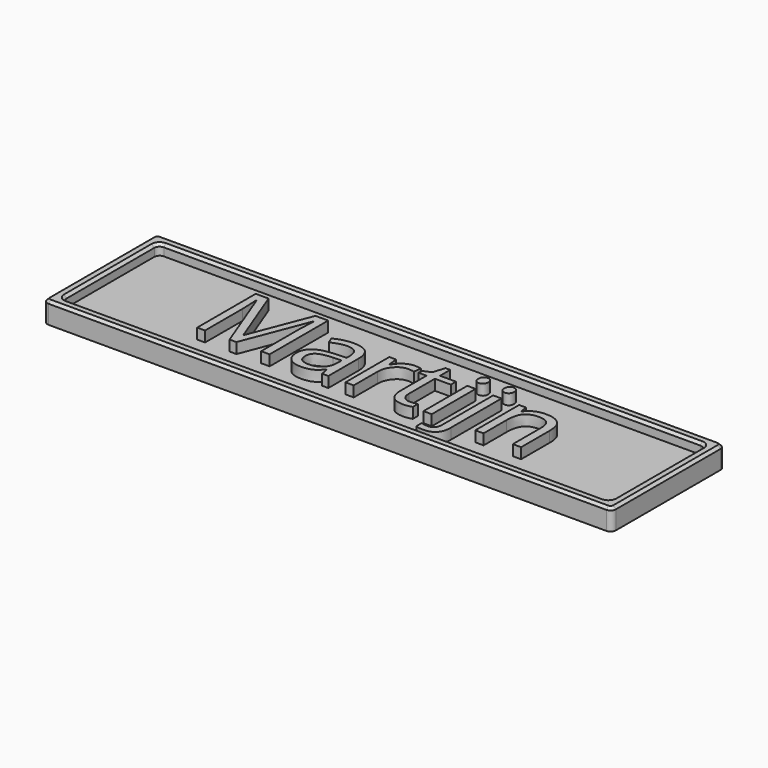
from build123d import *

# Parameters (mm, degrees)
F1_DEPTH     = 4
F0_TEXT_SIZE = 19.3397863768
F2_DEPTH     = 4
F0_W         = 1.5683358015
F0_H         = 10.3498075532
F3_DEPTH     = 2
F4_SIZE      = 0.5


# Not quite as in the source:
# - Text() gives the source's letters only with a copy of the font that has no kerning and outlines rounded to 1/6400 em; it was checked with that copy


with BuildPart() as f1:
    # F0 (on Top) → F1 (new body)
    with BuildSketch(Plane.XY):
        with BuildLine():
            Line((-52.6345206201, -13.340712525), (52.6345206201, -13.340712525))
            ThreePointArc((52.6345206201, -13.340712525), (53.3416274013, -13.0478193061), (53.6345206201, -12.340712525))
            Line((53.6345206201, -12.340712525), (53.6345206201, 12.340712525))
            ThreePointArc((53.6345206201, 12.340712525), (53.3416274013, 13.0478193061), (52.6345206201, 13.340712525))
            Line((52.6345206201, 13.340712525), (32.1950025846, 13.340712525))
            Line((32.1950025846, 13.340712525), (-52.6345206201, 13.340712525))
            ThreePointArc((-52.6345206201, 13.340712525), (-53.3416274013, 13.0478193061), (-53.6345206201, 12.340712525))
            Line((-53.6345206201, 12.340712525), (-53.6345206201, -12.340712525))
            ThreePointArc((-53.6345206201, -12.340712525), (-53.3416274013, -13.0478193061), (-52.6345206201, -13.340712525))
        make_face()
        with BuildLine():
            Line((-50.6345206201, 11.340712525), (50.6345206201, 11.340712525))
            ThreePointArc((50.6345206201, 11.340712525), (51.3416274013, 11.0478193061), (51.6345206201, 10.340712525))
            Line((51.6345206201, 10.340712525), (51.6345206201, -10.340712525))
            ThreePointArc((51.6345206201, -10.340712525), (51.3416274013, -11.0478193061), (50.6345206201, -11.340712525))
            Line((50.6345206201, -11.340712525), (-50.6345206201, -11.340712525))
            ThreePointArc((-50.6345206201, -11.340712525), (-51.3416274013, -11.0478193061), (-51.6345206201, -10.340712525))
            Line((-51.6345206201, -10.340712525), (-51.6345206201, 10.340712525))
            ThreePointArc((-51.6345206201, 10.340712525), (-51.3416274013, 11.0478193061), (-50.6345206201, 11.340712525))
        make_face(mode=Mode.SUBTRACT)
    extrude(amount=F1_DEPTH)



with BuildPart() as f2:
    # F0 (on Top) → F2 (new body)
    with BuildSketch(Plane.XY):
        with Locations((-32.0946779102, -6.3302232884)):
            Text('Martijn', F0_TEXT_SIZE, font='Open Sans', text_align=(TextAlign.LEFT, TextAlign.BOTTOM))
    extrude(amount=F2_DEPTH)


with BuildPart() as f1_1:
    add(f1.part)

    add(f2.part)  # F3 merges F2
    # F0 (on Top) → F3 (join)
    with BuildSketch(Plane.XY):
        with BuildLine():
            ThreePointArc((51.6345206201, 10.340712525), (51.3416274013, 11.0478193061), (50.6345206201, 11.340712525))
            Line((50.6345206201, 11.340712525), (-50.6345206201, 11.340712525))
            ThreePointArc((-50.6345206201, 11.340712525), (-51.3416274013, 11.0478193061), (-51.6345206201, 10.340712525))
            Line((-51.6345206201, 10.340712525), (-51.6345206201, -10.340712525))
            ThreePointArc((-51.6345206201, -10.340712525), (-51.3416274013, -11.0478193061), (-50.6345206201, -11.340712525))
            Line((-50.6345206201, -11.340712525), (50.6345206201, -11.340712525))
            ThreePointArc((50.6345206201, -11.340712525), (51.3416274013, -11.0478193061), (51.6345206201, -10.340712525))
            Line((51.6345206201, -10.340712525), (51.6345206201, 10.340712525))
        make_face()
        with BuildLine():
            Line((-5.4450566513, -6.3302232884), (-6.6084656755, -6.3302232884))
            Line((-6.6084656755, -6.3302232884), (-6.9197153625, -4.8555645772))
            Line((-6.9197153625, -4.8555645772), (-6.9952614031, -4.8555645772))
            add(Edge.make_bspline(
                [(-6.9952614031, -4.8555645772), (-7.7688528581, -5.8285975792), (-8.5379115508, -6.1745984449)],
                knots=[0, 0, 0, 1, 1, 1], degree=2))
            add(Edge.make_bspline(
                [(-8.5379115508, -6.1745984449), (-9.3069702434, -6.5205993105), (-10.4613137428, -6.5205993105)],
                knots=[0, 0, 0, 1, 1, 1], degree=2))
            add(Edge.make_bspline(
                [(-10.4613137428, -6.5205993105), (-11.9994311281, -6.5205993105), (-12.8727433566, -5.7258549641)],
                knots=[0, 0, 0, 1, 1, 1], degree=2))
            add(Edge.make_bspline(
                [(-12.8727433566, -5.7258549641), (-13.7460555852, -4.9311106177), (-13.7460555852, -3.4685392729)],
                knots=[0, 0, 0, 1, 1, 1], degree=2))
            add(Edge.make_bspline(
                [(-13.7460555852, -3.4685392729), (-13.7460555852, -0.3348895116), (-8.7328203354, -0.1837974305)],
                knots=[0, 0, 0, 1, 1, 1], degree=2))
            Line((-8.7328203354, -0.1837974305), (-6.9771303533, -0.1263824397))
            Line((-6.9771303533, -0.1263824397), (-6.9771303533, 0.5172698257))
            add(Edge.make_bspline(
                [(-6.9771303533, 0.5172698257), (-6.9771303533, 1.7350719991), (-7.4999089538, 2.3152655904)],
                knots=[0, 0, 0, 1, 1, 1], degree=2))
            add(Edge.make_bspline(
                [(-7.4999089538, 2.3152655904), (-8.0226875543, 2.8954591817), (-9.1770310537, 2.8954591817)],
                knots=[0, 0, 0, 1, 1, 1], degree=2))
            add(Edge.make_bspline(
                [(-9.1770310537, 2.8954591817), (-10.4703792676, 2.8954591817), (-12.1021737432, 2.1037366769)],
                knots=[0, 0, 0, 1, 1, 1], degree=2))
            Line((-12.1021737432, 2.1037366769), (-12.5856684026, 3.3034078006))
            add(Edge.make_bspline(
                [(-12.5856684026, 3.3034078006), (-11.8211424724, 3.7174001027), (-10.9100572236, 3.9531037492)],
                knots=[0, 0, 0, 1, 1, 1], degree=2))
            add(Edge.make_bspline(
                [(-10.9100572236, 3.9531037492), (-9.9989719747, 4.1888073956), (-9.0803321218, 4.1888073956)],
                knots=[0, 0, 0, 1, 1, 1], degree=2))
            add(Edge.make_bspline(
                [(-9.0803321218, 4.1888073956), (-7.2309650495, 4.1888073956), (-6.3380108504, 3.3683773954)],
                knots=[0, 0, 0, 1, 1, 1], degree=2))
            add(Edge.make_bspline(
                [(-6.3380108504, 3.3683773954), (-5.4450566513, 2.5479473952), (-5.4450566513, 0.7348424224)],
                knots=[0, 0, 0, 1, 1, 1], degree=2))
            Line((-5.4450566513, 0.7348424224), (-5.4450566513, -6.3302232884))
        make_face(mode=Mode.SUBTRACT)
        with BuildLine():
            add(Edge.make_bspline(
                [(18.9653799662, -7.9166901396), (18.9653799662, -10.9778157021), (16.1399580502, -10.9778157021)],
                knots=[0, 0, 0, 1, 1, 1], degree=2))
            add(Edge.make_bspline(
                [(16.1399580502, -10.9778157021), (15.2424710886, -10.9778157021), (14.6864522303, -10.739090214)],
                knots=[0, 0, 0, 1, 1, 1], degree=2))
            Line((14.6864522303, -10.739090214), (14.6864522303, -9.4668948914))
            add(Edge.make_bspline(
                [(14.6864522303, -9.4668948914), (15.3391700205, -9.6542490719), (15.9707349194, -9.6542490719)],
                knots=[0, 0, 0, 1, 1, 1], degree=2))
            add(Edge.make_bspline(
                [(15.9707349194, -9.6542490719), (16.708064275, -9.6542490719), (17.0525542198, -9.2523441363)],
                knots=[0, 0, 0, 1, 1, 1], degree=2))
            add(Edge.make_bspline(
                [(17.0525542198, -9.2523441363), (17.3970441647, -8.8504392006), (17.3970441647, -8.0315201212)],
                knots=[0, 0, 0, 1, 1, 1], degree=2))
            Line((17.3970441647, -8.0315201212), (17.3970441647, 4.0195842648))
            Line((17.3970441647, 4.0195842648), (18.9653799662, 4.0195842648))
            Line((18.9653799662, 4.0195842648), (18.9653799662, -7.9166901396))
        make_face(mode=Mode.SUBTRACT)
        with BuildLine():
            add(Edge.make_bspline(
                [(0.7195002563, 3.6614960327), (1.5323756525, 4.209960287), (2.5054086545, 4.209960287)],
                knots=[0, 0, 0, 1, 1, 1], degree=2))
            add(Edge.make_bspline(
                [(2.5054086545, 4.209960287), (3.1943885442, 4.209960287), (3.7413418777, 4.0951303054)],
                knots=[0, 0, 0, 1, 1, 1], degree=2))
            Line((3.7413418777, 4.0951303054), (3.5237692809, 2.6416244855))
            add(Edge.make_bspline(
                [(3.5237692809, 2.6416244855), (2.8831388572, 2.7836510417), (2.3905786729, 2.7836510417)],
                knots=[0, 0, 0, 1, 1, 1], degree=2))
            add(Edge.make_bspline(
                [(2.3905786729, 2.7836510417), (1.1334925584, 2.7836510417), (0.2420492801, 1.7637794945)],
                knots=[0, 0, 0, 1, 1, 1], degree=2))
            add(Edge.make_bspline(
                [(0.2420492801, 1.7637794945), (-0.6493939982, 0.7439079473), (-0.6493939982, -0.7760783883)],
                knots=[0, 0, 0, 1, 1, 1], degree=2))
            Line((-0.6493939982, -0.7760783883), (-0.6493939982, -6.3302232884))
            Line((-0.6493939982, -6.3302232884), (-2.2177297997, -6.3302232884))
            Line((-2.2177297997, -6.3302232884), (-2.2177297997, 4.0195842648))
            Line((-2.2177297997, 4.0195842648), (-0.9243815857, 4.0195842648))
            Line((-0.9243815857, 4.0195842648), (-0.7430710884, 2.1037366769))
            Line((-0.7430710884, 2.1037366769), (-0.6675250479, 2.1037366769))
            add(Edge.make_bspline(
                [(-0.6675250479, 2.1037366769), (-0.0933751398, 3.1130317784), (0.7195002563, 3.6614960327)],
                knots=[0, 0, 0, 1, 1, 1], degree=2))
        make_face(mode=Mode.SUBTRACT)
        with Locations((13.2888504804, -1.1553195118)):
            Rectangle(F0_W, F0_H, mode=Mode.SUBTRACT)
        with BuildLine():
            add(Edge.make_bspline(
                [(7.8026970168, -4.7241144666), (8.2469077352, -5.224229255), (9.0204991902, -5.224229255)],
                knots=[0, 0, 0, 1, 1, 1], degree=2))
            add(Edge.make_bspline(
                [(9.0204991902, -5.224229255), (9.437513334, -5.224229255), (9.8243090615, -5.1637924225)],
                knots=[0, 0, 0, 1, 1, 1], degree=2))
            add(Edge.make_bspline(
                [(9.8243090615, -5.1637924225), (10.2111047891, -5.1033555901), (10.4377429107, -5.0368750744)],
                knots=[0, 0, 0, 1, 1, 1], degree=2))
            Line((10.4377429107, -5.0368750744), (10.4377429107, -6.2365461981))
            add(Edge.make_bspline(
                [(10.4377429107, -6.2365461981), (10.1839082145, -6.357419863), (9.6883261886, -6.4390095868)],
                knots=[0, 0, 0, 1, 1, 1], degree=2))
            add(Edge.make_bspline(
                [(9.6883261886, -6.4390095868), (9.1927441626, -6.5205993105), (8.7938610686, -6.5205993105)],
                knots=[0, 0, 0, 1, 1, 1], degree=2))
            add(Edge.make_bspline(
                [(8.7938610686, -6.5205993105), (5.7931723386, -6.5205993105), (5.7931723386, -3.356731133)],
                knots=[0, 0, 0, 1, 1, 1], degree=2))
            Line((5.7931723386, -3.356731133), (5.7931723386, 2.8017820914))
            Line((5.7931723386, 2.8017820914), (4.3094481025, 2.8017820914))
            Line((4.3094481025, 2.8017820914), (4.3094481025, 3.5572424968))
            Line((4.3094481025, 3.5572424968), (5.7931723386, 4.209960287))
            Line((5.7931723386, 4.209960287), (6.4519338121, 6.4189265122))
            Line((6.4519338121, 6.4189265122), (7.3584862985, 6.4189265122))
            Line((7.3584862985, 6.4189265122), (7.3584862985, 4.0195842648))
            Line((7.3584862985, 4.0195842648), (10.3621968701, 4.0195842648))
            Line((10.3621968701, 4.0195842648), (10.3621968701, 2.8017820914))
            Line((10.3621968701, 2.8017820914), (7.3584862985, 2.8017820914))
            Line((7.3584862985, 2.8017820914), (7.3584862985, -3.2902506173))
            add(Edge.make_bspline(
                [(7.3584862985, -3.2902506173), (7.3584862985, -4.2239996783), (7.8026970168, -4.7241144666)],
                knots=[0, 0, 0, 1, 1, 1], degree=2))
        make_face(mode=Mode.SUBTRACT)
        with BuildLine():
            Line((30.9409383117, -6.3302232884), (29.3726025102, -6.3302232884))
            Line((29.3726025102, -6.3302232884), (29.3726025102, 0.3661777446))
            add(Edge.make_bspline(
                [(29.3726025102, 0.3661777446), (29.3726025102, 1.6293075423), (28.7969416813, 2.2533178371)],
                knots=[0, 0, 0, 1, 1, 1], degree=2))
            add(Edge.make_bspline(
                [(28.7969416813, 2.2533178371), (28.2212808524, 2.8773281319), (26.9913913125, 2.8773281319)],
                knots=[0, 0, 0, 1, 1, 1], degree=2))
            add(Edge.make_bspline(
                [(26.9913913125, 2.8773281319), (25.3686623619, 2.8773281319), (24.6132019565, 1.9994831409)],
                knots=[0, 0, 0, 1, 1, 1], degree=2))
            add(Edge.make_bspline(
                [(24.6132019565, 1.9994831409), (23.8577415512, 1.1216381499), (23.8577415512, -0.8999738948)],
                knots=[0, 0, 0, 1, 1, 1], degree=2))
            Line((23.8577415512, -0.8999738948), (23.8577415512, -6.3302232884))
            Line((23.8577415512, -6.3302232884), (22.2894057497, -6.3302232884))
            Line((22.2894057497, -6.3302232884), (22.2894057497, 4.0195842648))
            Line((22.2894057497, 4.0195842648), (23.5646229139, 4.0195842648))
            Line((23.5646229139, 4.0195842648), (23.8184576101, 2.6023405444))
            Line((23.8184576101, 2.6023405444), (23.8940036506, 2.6023405444))
            add(Edge.make_bspline(
                [(23.8940036506, 2.6023405444), (24.3774983101, 3.3668664746), (25.2462777762, 3.7884133808)],
                knots=[0, 0, 0, 1, 1, 1], degree=2))
            add(Edge.make_bspline(
                [(25.2462777762, 3.7884133808), (26.1150572424, 4.209960287), (27.1817673347, 4.209960287)],
                knots=[0, 0, 0, 1, 1, 1], degree=2))
            add(Edge.make_bspline(
                [(27.1817673347, 4.209960287), (29.0522872983, 4.209960287), (29.996612805, 3.307940563)],
                knots=[0, 0, 0, 1, 1, 1], degree=2))
            add(Edge.make_bspline(
                [(29.996612805, 3.307940563), (30.9409383117, 2.405920839), (30.9409383117, 0.4205708938)],
                knots=[0, 0, 0, 1, 1, 1], degree=2))
            Line((30.9409383117, 0.4205708938), (30.9409383117, -6.3302232884))
        make_face(mode=Mode.SUBTRACT)
        with BuildLine():
            Line((-22.7934493996, -6.3302232884), (-24.0867976136, -6.3302232884))
            Line((-24.0867976136, -6.3302232884), (-28.7706521267, 5.9082352782))
            Line((-28.7706521267, 5.9082352782), (-28.8461981672, 5.9082352782))
            add(Edge.make_bspline(
                [(-28.8461981672, 5.9082352782), (-28.7132371359, 4.4547294583), (-28.7132371359, 2.4512484633)],
                knots=[0, 0, 0, 1, 1, 1], degree=2))
            Line((-28.7132371359, 2.4512484633), (-28.7132371359, -6.3302232884))
            Line((-28.7132371359, -6.3302232884), (-30.196961372, -6.3302232884))
            Line((-30.196961372, -6.3302232884), (-30.196961372, 7.4765710797))
            Line((-30.196961372, 7.4765710797), (-27.7794880749, 7.4765710797))
            Line((-27.7794880749, 7.4765710797), (-23.4068832488, -3.9127499913))
            Line((-23.4068832488, -3.9127499913), (-23.3313372082, -3.9127499913))
            Line((-23.3313372082, -3.9127499913), (-18.9224702826, 7.4765710797))
            Line((-18.9224702826, 7.4765710797), (-16.5231280353, 7.4765710797))
            Line((-16.5231280353, 7.4765710797), (-16.5231280353, -6.3302232884))
            Line((-16.5231280353, -6.3302232884), (-18.1277259362, -6.3302232884))
            Line((-18.1277259362, -6.3302232884), (-18.1277259362, 2.5660784449))
            add(Edge.make_bspline(
                [(-18.1277259362, 2.5660784449), (-18.1277259362, 4.0951303054), (-17.9947649049, 5.8901042285)],
                knots=[0, 0, 0, 1, 1, 1], degree=2))
            Line((-17.9947649049, 5.8901042285), (-18.0703109454, 5.8901042285))
            Line((-18.0703109454, 5.8901042285), (-22.7934493996, -6.3302232884))
        make_face(mode=Mode.SUBTRACT)
        with BuildLine():
            add(Edge.make_bspline(
                [(12.6361326902, 6.0351526263), (12.3717215483, 6.2950310057), (12.3717215483, 6.8238532895)],
                knots=[0, 0, 0, 1, 1, 1], degree=2))
            add(Edge.make_bspline(
                [(12.3717215483, 6.8238532895), (12.3717215483, 7.3617410981), (12.6361326902, 7.6125539526)],
                knots=[0, 0, 0, 1, 1, 1], degree=2))
            add(Edge.make_bspline(
                [(12.6361326902, 7.6125539526), (12.9005438321, 7.8633668072), (13.2994269261, 7.8633668072)],
                knots=[0, 0, 0, 1, 1, 1], degree=2))
            add(Edge.make_bspline(
                [(13.2994269261, 7.8633668072), (13.6771571288, 7.8633668072), (13.9506337955, 7.6080211902)],
                knots=[0, 0, 0, 1, 1, 1], degree=2))
            add(Edge.make_bspline(
                [(13.9506337955, 7.6080211902), (14.2241104622, 7.3526755732), (14.2241104622, 6.8238532895)],
                knots=[0, 0, 0, 1, 1, 1], degree=2))
            add(Edge.make_bspline(
                [(14.2241104622, 6.8238532895), (14.2241104622, 6.2950310057), (13.9506337955, 6.0351526263)],
                knots=[0, 0, 0, 1, 1, 1], degree=2))
            add(Edge.make_bspline(
                [(13.9506337955, 6.0351526263), (13.6771571288, 5.7752742468), (13.2994269261, 5.7752742468)],
                knots=[0, 0, 0, 1, 1, 1], degree=2))
            add(Edge.make_bspline(
                [(13.2994269261, 5.7752742468), (12.9005438321, 5.7752742468), (12.6361326902, 6.0351526263)],
                knots=[0, 0, 0, 1, 1, 1], degree=2))
        make_face(mode=Mode.SUBTRACT)
        with BuildLine():
            add(Edge.make_bspline(
                [(17.5284942752, 6.0351526263), (17.2640831333, 6.2950310057), (17.2640831333, 6.8238532895)],
                knots=[0, 0, 0, 1, 1, 1], degree=2))
            add(Edge.make_bspline(
                [(17.2640831333, 6.8238532895), (17.2640831333, 7.3617410981), (17.5284942752, 7.6125539526)],
                knots=[0, 0, 0, 1, 1, 1], degree=2))
            add(Edge.make_bspline(
                [(17.5284942752, 7.6125539526), (17.7929054171, 7.8633668072), (18.1917885111, 7.8633668072)],
                knots=[0, 0, 0, 1, 1, 1], degree=2))
            add(Edge.make_bspline(
                [(18.1917885111, 7.8633668072), (18.5695187138, 7.8633668072), (18.8429953805, 7.6080211902)],
                knots=[0, 0, 0, 1, 1, 1], degree=2))
            add(Edge.make_bspline(
                [(18.8429953805, 7.6080211902), (19.1164720472, 7.3526755732), (19.1164720472, 6.8238532895)],
                knots=[0, 0, 0, 1, 1, 1], degree=2))
            add(Edge.make_bspline(
                [(19.1164720472, 6.8238532895), (19.1164720472, 6.2950310057), (18.8429953805, 6.0351526263)],
                knots=[0, 0, 0, 1, 1, 1], degree=2))
            add(Edge.make_bspline(
                [(18.8429953805, 6.0351526263), (18.5695187138, 5.7752742468), (18.1917885111, 5.7752742468)],
                knots=[0, 0, 0, 1, 1, 1], degree=2))
            add(Edge.make_bspline(
                [(18.1917885111, 5.7752742468), (17.7929054171, 5.7752742468), (17.5284942752, 6.0351526263)],
                knots=[0, 0, 0, 1, 1, 1], degree=2))
        make_face(mode=Mode.SUBTRACT)
        with BuildLine():
            add(Edge.make_bspline(
                [(-11.5884606676, -4.7815294574), (-11.0747475919, -5.224229255), (-10.1500640558, -5.224229255)],
                knots=[0, 0, 0, 1, 1, 1], degree=2))
            add(Edge.make_bspline(
                [(-10.1500640558, -5.224229255), (-8.6844708694, -5.224229255), (-7.8489316611, -4.4219303045)],
                knots=[0, 0, 0, 1, 1, 1], degree=2))
            add(Edge.make_bspline(
                [(-7.8489316611, -4.4219303045), (-7.0133924528, -3.619631354), (-7.0133924528, -2.175191059)],
                knots=[0, 0, 0, 1, 1, 1], degree=2))
            Line((-7.0133924528, -2.175191059), (-7.0133924528, -1.241441998))
            Line((-7.0133924528, -1.241441998), (-8.5817282543, -1.304900672))
            add(Edge.make_bspline(
                [(-8.5817282543, -1.304900672), (-10.4522482179, -1.3713811877), (-11.2772109806, -1.8866051842)],
                knots=[0, 0, 0, 1, 1, 1], degree=2))
            add(Edge.make_bspline(
                [(-11.2772109806, -1.8866051842), (-12.1021737432, -2.4018291806), (-12.1021737432, -3.4866703227)],
                knots=[0, 0, 0, 1, 1, 1], degree=2))
            add(Edge.make_bspline(
                [(-12.1021737432, -3.4866703227), (-12.1021737432, -4.3388296599), (-11.5884606676, -4.7815294574)],
                knots=[0, 0, 0, 1, 1, 1], degree=2))
        make_face()
    extrude(amount=F3_DEPTH)

    # F4
    f4_edges = [f1_1.edges().sort_by_distance(p)[0] for p in [
        (0, 13.340713, 4),
        (-53.341627, 13.047819, 4),
        (-53.634521, 0, 4),
        (0, -13.340713, 4),
        (-53.341627, -13.047819, 4),
        (0, 11.340713, 4),
    ]]
    chamfer(f4_edges, length=F4_SIZE)


solid = f1_1.part
